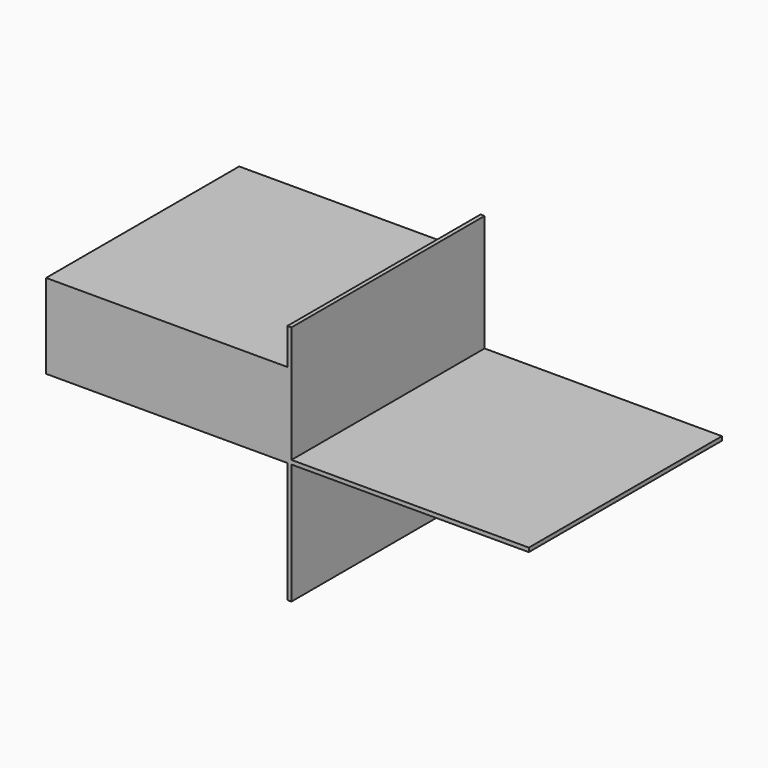
from build123d import *

# Parameters (mm, degrees)
F0_W     = 600
F0_H     = 300
F1_DEPTH = 5
F2_W     = 300
F2_H     = 300
F3_DEPTH = 5
F6_W     = 300
F6_H     = 300
F7_DEPTH = 100


# Not quite as in the source:
# - the program builds the solid bodies; features that only make, move or delete a surface that nothing else refers to are left out


with BuildPart() as f1:
    # F0 (on Top) → F1 (new body)
    with BuildSketch(Plane.XY):
        Rectangle(F0_W, F0_H)
    extrude(amount=F1_DEPTH)

    # F2 (on Right) → F3 (join)
    with BuildSketch(Plane.YZ):
        Rectangle(F2_W, F2_H)
    extrude(amount=F3_DEPTH)

    # F6 (on face) → F7 (join)
    with BuildSketch(Plane.XY.offset(5)):
        with Locations((-150, 0)):
            Rectangle(F6_W, F6_H)
    extrude(amount=F7_DEPTH)


solid = f1.part
